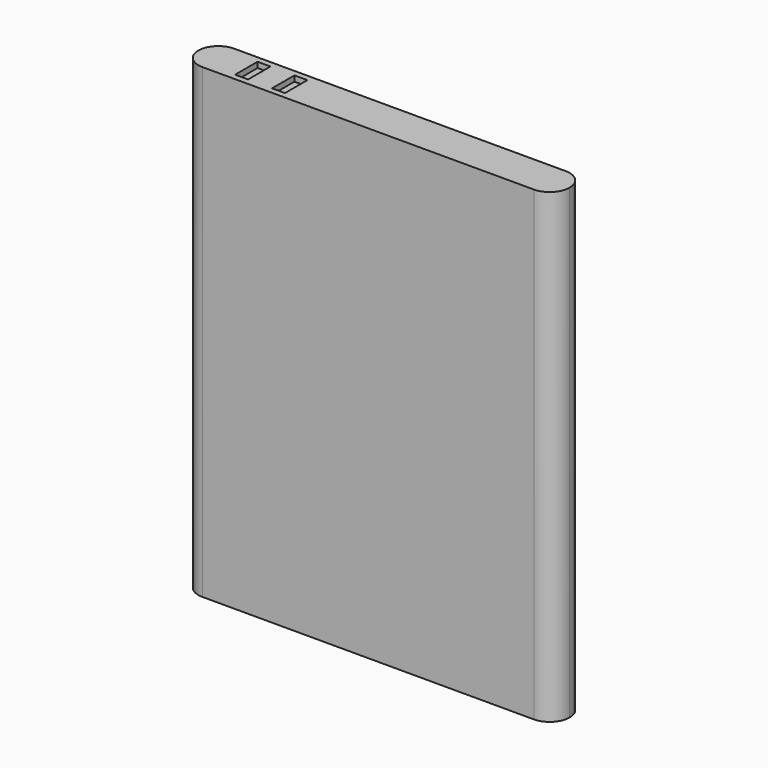
from build123d import *

# Parameters (mm, degrees)
F0_W     = 50.3
F0_H     = 63.2
F1_DEPTH = 2.7
F2_R     = 2.69999
F3_W     = 1.75
F3_H     = 3.8
F4_DEPTH = 0.75


# Not quite as in the source:
# - a fillet or chamfer is up to 0.001 mm smaller than in the source, because OpenCascade refuses the exact size


with BuildPart() as f1:
    # F0 (on Front) → F1 (new body, symmetric)
    with BuildSketch(Plane.XZ):
        Rectangle(F0_W, F0_H)
    extrude(amount=F1_DEPTH, both=True)

    # F2 (radius 2.7 in the source; OpenCascade refuses exactly that, so slightly less here)
    f2_edges = [f1.edges().sort_by_distance(p)[0] for p in [
        (25.15, 2.7, 0),
        (25.15, -2.7, 0),
        (-25.15, -2.7, 0),
        (-25.15, 2.7, 0),
    ]]
    fillet(f2_edges, radius=F2_R)

    # F3 (on face) → F4 (cut)
    with BuildSketch(Plane.XY.offset(31.6)):
        with Locations((-17.775, 0)):
            Rectangle(F3_W, F3_H)
        with Locations((-12.775, 0)):
            Rectangle(F3_W, F3_H)
    extrude(amount=-F4_DEPTH, mode=Mode.SUBTRACT)


solid = f1.part
